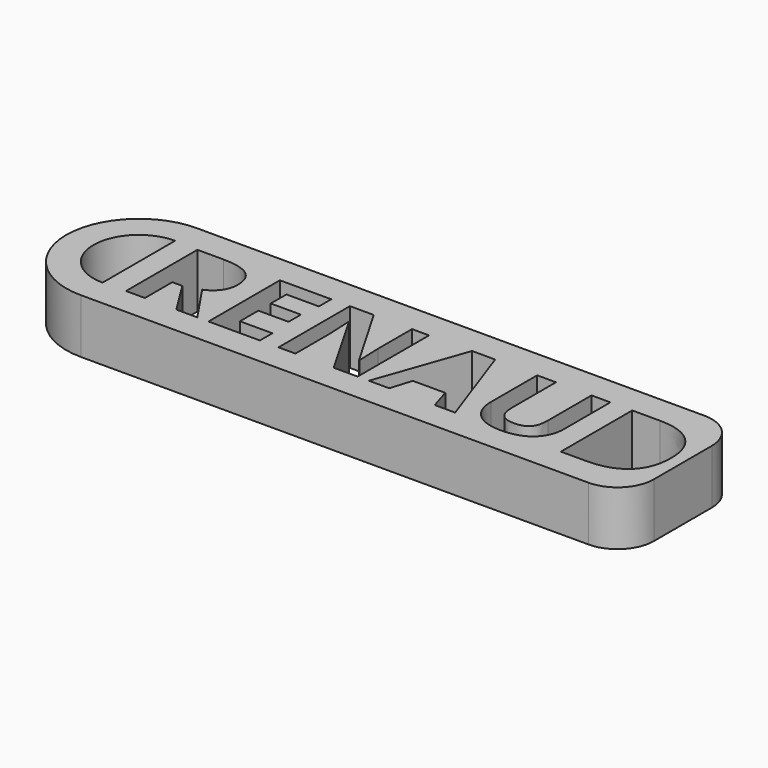
from build123d import *

# Parameters (mm, degrees)
F1_DEPTH = 3


# Not quite as in the source:
# - a feature names something its author has since deleted; it is built from what else it names


with BuildPart() as f1:
    # F0 (on Top) → F1 (new body)
    with BuildSketch(Plane.XY):
        with BuildLine():
            Line((-15, 2.5), (-15, 4))
            ThreePointArc((-15, 4), (-19, 0), (-15, -4))
            Line((-15, -4), (-15, -2.5))
            ThreePointArc((-15, -2.5), (-17.5, 0), (-15, 2.5))
        make_face()
        with BuildLine():
            Line((13, 4), (-15, 4))
            Line((-15, 4), (-15, 2.5))
            Line((-15, 2.5), (-15, -2.5))
            Line((-15, -2.5), (-15, -4))
            Line((-15, -4), (13, -4))
            ThreePointArc((13, -4), (14.4142135624, -3.4142135624), (15, -2))
            Line((15, -2), (15, 2))
            ThreePointArc((15, 2), (14.4142135624, 3.4142135624), (13, 4))
        make_face()
        with BuildLine():
            Line((-12.1249144637, -0.5934820884), (-12.6796209529, -0.5934820884))
            Line((-12.6796209529, -0.5934820884), (-12.6796209529, -2.4816383516))
            Line((-12.6796209529, -2.4816383516), (-13.7233308326, -2.4816383516))
            Line((-13.7233308326, -2.4816383516), (-13.7233308326, 2.4396314525))
            Line((-13.7233308326, 2.4396314525), (-12.2897107605, 2.4396314525))
            add(Edge.make_bspline(
                [(-12.2897107605, 2.4396314525), (-11.2858535801, 2.4396314525), (-10.8049284394, 2.0744945596)],
                knots=[0, 0, 0, 1, 1, 1], degree=2))
            add(Edge.make_bspline(
                [(-10.8049284394, 2.0744945596), (-10.3240032988, 1.7093576667), (-10.3240032988, 0.9650815812)],
                knots=[0, 0, 0, 1, 1, 1], degree=2))
            add(Edge.make_bspline(
                [(-10.3240032988, 0.9650815812), (-10.3240032988, 0.5310102897), (-10.5625809441, 0.1928008962)],
                knots=[0, 0, 0, 1, 1, 1], degree=2))
            add(Edge.make_bspline(
                [(-10.5625809441, 0.1928008962), (-10.8011585895, -0.1454084972), (-11.239538281, -0.3371322934)],
                knots=[0, 0, 0, 1, 1, 1], degree=2))
            add(Edge.make_bspline(
                [(-11.239538281, -0.3371322934), (-10.1279711026, -1.9969433611), (-9.7919159092, -2.4816383516)],
                knots=[0, 0, 0, 1, 1, 1], degree=2))
            Line((-9.7919159092, -2.4816383516), (-10.9497983866, -2.4816383516))
            Line((-10.9497983866, -2.4816383516), (-12.1249144637, -0.5934820884))
        make_face(mode=Mode.SUBTRACT)
        Polygon((-6.3387333765, -1.6199583684), (-6.3387333765, -2.4816383516), (-9.1725834212, -2.4816383516), (-9.1725834212, 2.4396314525), (-6.3387333765, 2.4396314525), (-6.3387333765, 1.5844140691), (-8.1288735416, 1.5844140691), (-8.1288735416, 0.5040827902), (-6.4625998741, 0.5040827902), (-6.4625998741, -0.3511345932), (-8.1288735416, -0.3511345932), (-8.1288735416, -1.6199583684), align=None, mode=Mode.SUBTRACT)
        with BuildLine():
            Line((-0.9467708815, 2.4396314525), (-0.9467708815, -2.4816383516))
            Line((-0.9467708815, -2.4816383516), (-2.2726809557, -2.4816383516))
            Line((-2.2726809557, -2.4816383516), (-4.413955714, 1.2408191758))
            Line((-4.413955714, 1.2408191758), (-4.4441145134, 1.2408191758))
            add(Edge.make_bspline(
                [(-4.4441145134, 1.2408191758), (-4.3794885146, 0.255272695), (-4.3794885146, -0.1658733968)],
                knots=[0, 0, 0, 1, 1, 1], degree=2))
            Line((-4.3794885146, -0.1658733968), (-4.3794885146, -2.4816383516))
            Line((-4.3794885146, -2.4816383516), (-5.3122570965, -2.4816383516))
            Line((-5.3122570965, -2.4816383516), (-5.3122570965, 2.4396314525))
            Line((-5.3122570965, 2.4396314525), (-3.9960409221, 2.4396314525))
            Line((-3.9960409221, 2.4396314525), (-1.8590745638, -1.2462046757))
            Line((-1.8590745638, -1.2462046757), (-1.8353783642, -1.2462046757))
            add(Edge.make_bspline(
                [(-1.8353783642, -1.2462046757), (-1.8860020632, -0.2865085944), (-1.8860020632, 0.1098641979)],
                knots=[0, 0, 0, 1, 1, 1], degree=2))
            Line((-1.8860020632, 0.1098641979), (-1.8860020632, 2.4396314525))
            Line((-1.8860020632, 2.4396314525), (-0.9467708815, 2.4396314525))
        make_face(mode=Mode.SUBTRACT)
        Polygon((4.4290351137, -2.4816383516), (3.3045427356, -2.4816383516), (2.9480226425, -1.3097535745), (1.1535740775, -1.3097535745), (0.7970539845, -2.4816383516), (-0.3274383936, -2.4816383516), (1.4099238725, 2.4600963521), (2.6852102477, 2.4600963521), align=None, mode=Mode.SUBTRACT)
        with BuildLine():
            Line((8.0136238438, 2.4396314525), (9.0541024235, 2.4396314525))
            Line((9.0541024235, 2.4396314525), (9.0541024235, -0.7442760855))
            add(Edge.make_bspline(
                [(9.0541024235, -0.7442760855), (9.0541024235, -1.2903657749), (8.8101392783, -1.7007408669)],
                knots=[0, 0, 0, 1, 1, 1], degree=2))
            add(Edge.make_bspline(
                [(8.8101392783, -1.7007408669), (8.5661761331, -2.1111159589), (8.1046387921, -2.3303058046)],
                knots=[0, 0, 0, 1, 1, 1], degree=2))
            add(Edge.make_bspline(
                [(8.1046387921, -2.3303058046), (7.643101451, -2.5494956503), (7.0140750633, -2.5494956503)],
                knots=[0, 0, 0, 1, 1, 1], degree=2))
            add(Edge.make_bspline(
                [(7.0140750633, -2.5494956503), (6.0651499818, -2.5494956503), (5.540063742, -2.0626464598)],
                knots=[0, 0, 0, 1, 1, 1], degree=2))
            add(Edge.make_bspline(
                [(5.540063742, -2.0626464598), (5.0149775023, -1.5757972693), (5.0149775023, -0.7313508857)],
                knots=[0, 0, 0, 1, 1, 1], degree=2))
            Line((5.0149775023, -0.7313508857), (5.0149775023, 2.4396314525))
            Line((5.0149775023, 2.4396314525), (6.054378982, 2.4396314525))
            Line((6.054378982, 2.4396314525), (6.054378982, -0.5730171888))
            add(Edge.make_bspline(
                [(6.054378982, -0.5730171888), (6.054378982, -1.1417259777), (6.2832627275, -1.4077696726)],
                knots=[0, 0, 0, 1, 1, 1], degree=2))
            add(Edge.make_bspline(
                [(6.2832627275, -1.4077696726), (6.5121464731, -1.6738133674), (7.0410025628, -1.6738133674)],
                knots=[0, 0, 0, 1, 1, 1], degree=2))
            add(Edge.make_bspline(
                [(7.0410025628, -1.6738133674), (7.5526250528, -1.6738133674), (7.7831244483, -1.4061540226)],
                knots=[0, 0, 0, 1, 1, 1], degree=2))
            add(Edge.make_bspline(
                [(7.7831244483, -1.4061540226), (8.0136238438, -1.1384946778), (8.0136238438, -0.566554589)],
                knots=[0, 0, 0, 1, 1, 1], degree=2))
            Line((8.0136238438, -0.566554589), (8.0136238438, 2.4396314525))
        make_face(mode=Mode.SUBTRACT)
        with BuildLine():
            add(Edge.make_bspline(
                [(13.6759384335, 1.8036039149), (14.3426633205, 1.1675763772), (14.3426633205, 0.0258503995)],
                knots=[0, 0, 0, 1, 1, 1], degree=2))
            add(Edge.make_bspline(
                [(14.3426633205, 0.0258503995), (14.3426633205, -1.1891183768), (13.650626584, -1.8353783642)],
                knots=[0, 0, 0, 1, 1, 1], degree=2))
            add(Edge.make_bspline(
                [(13.650626584, -1.8353783642), (12.9585898475, -2.4816383516), (11.6531446729, -2.4816383516)],
                knots=[0, 0, 0, 1, 1, 1], degree=2))
            Line((11.6531446729, -2.4816383516), (10.2593773001, -2.4816383516))
            Line((10.2593773001, -2.4816383516), (10.2593773001, 2.4396314525))
            Line((10.2593773001, 2.4396314525), (11.80393867, 2.4396314525))
            add(Edge.make_bspline(
                [(11.80393867, 2.4396314525), (13.0092135465, 2.4396314525), (13.6759384335, 1.8036039149)],
                knots=[0, 0, 0, 1, 1, 1], degree=2))
        make_face(mode=Mode.SUBTRACT)
    extrude(amount=F1_DEPTH)


solid = f1.part
